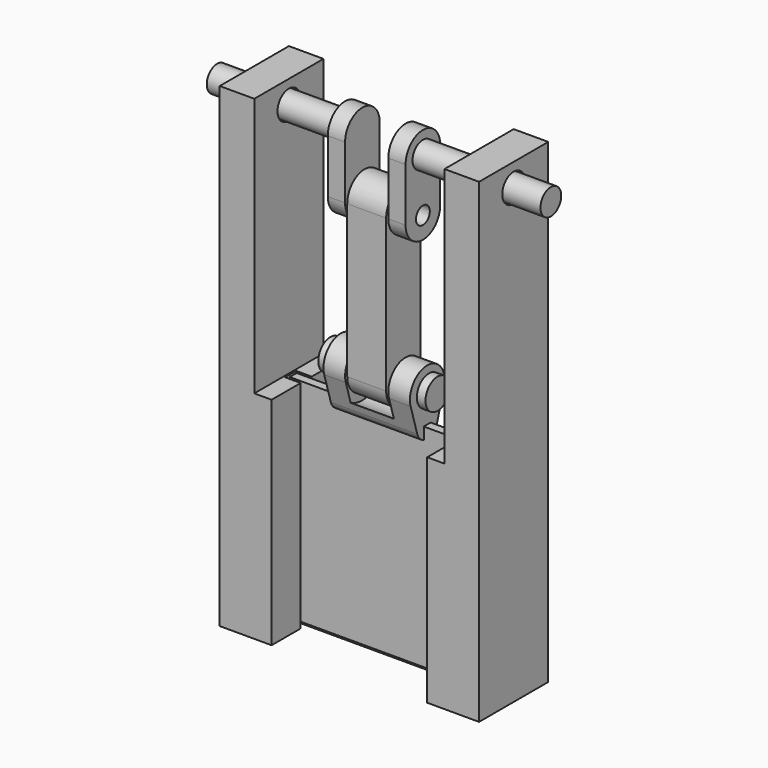
from build123d import *

# Parameters (mm, degrees)
F1_DEPTH  = 25
F0_W      = 21
F0_H      = 1
F2_SIZE   = 0.49999
F3_R      = 1
F4_DEPTH  = 5
F5_R      = 3.5
F5_R_2    = 1
F6_DEPTH  = 2.5
F7_R      = 0.8500000113
F8_DEPTH  = 5.2
F9_R      = 1.7489925994
F10_DEPTH = 1
F12_R     = 1
F12_R_2   = 1.1
F13_DEPTH = 2.25
F14_R     = 1
F15_DEPTH = 2.5
F16_R     = 1
F17_DEPTH = 2
F18_R     = 1.5
F19_DEPTH = 14.8
F21_W     = 10
F21_H     = 30
F21_R     = 1.65
F22_DEPTH = 4


# Not quite as in the source:
# - a fillet or chamfer is up to 0.001 mm smaller than in the source, because OpenCascade refuses the exact size


with BuildPart() as f1:
    # F0 (on Top) → F1 (new body)
    with BuildSketch(Plane.XY):
        Polygon((-9, 5), (-15, 5), (-15, -5), (-9, -5), (-9, -0.8), (-10.8, -0.8), (-10.8, 0.8), (-9, 0.8), align=None)
    extrude(amount=F1_DEPTH)

    # F23: F1b across plane


with BuildPart() as f1b:
    # F0 (on Top) → F1, piece 2 (new body)
    with BuildSketch(Plane.XY):
        Polygon((15, -5), (15, 5), (9, 5), (9, 0.8), (10.8, 0.8), (10.8, -0.8), (9, -0.8), (9, -5), align=None)
    extrude(amount=F1_DEPTH)

    # F21 (on face) → F22 (join)
    with BuildSketch(Plane.YZ.offset(15)):
        with Locations((0, 40)):
            Rectangle(F21_W, F21_H)
        with Locations((0, 52.3577854037)):
            Circle(F21_R, mode=Mode.SUBTRACT)
    extrude(amount=-F22_DEPTH)


with BuildPart() as f1c:
    # F0 (on Top) → F1, piece 3 (new body)
    with BuildSketch(Plane.XY):
        Rectangle(F0_W, F0_H)
    extrude(amount=F1_DEPTH)

    # F2 (size 0.5 in the source; OpenCascade refuses exactly that, so slightly less here)
    f2_edges = [f1c.edges().sort_by_distance(p)[0] for p in [
        (0, -0.5, 0),
        (0, 0.5, 0),
    ]]
    chamfer(f2_edges, length=F2_SIZE)

    # F3 (on Right) → F4 (join, symmetric)
    with BuildSketch(Plane.YZ):
        with BuildLine():
            Line((-2.3955912057, 27.8127531877), (-1.4373557878, 24.6019490366))
            ThreePointArc((-1.4373557878, 24.6019490366), (0, 23.5309109688), (1.4373557878, 24.6019490366))
            Line((1.4373557878, 24.6019490366), (2.3955912057, 27.8127531877))
            ThreePointArc((2.3955912057, 27.8127531877), (0, 31.0276956856), (-2.3955912057, 27.8127531877))
        make_face()
        with Locations((0, 28.5276956856)):
            Circle(F3_R, mode=Mode.SUBTRACT)
    extrude(amount=F4_DEPTH, both=True)

    # F5 (on Right) → F6 (cut, symmetric)
    with BuildSketch(Plane.YZ):
        with Locations((0, 28.5276956856)):
            Circle(F5_R)
        with Locations((0, 28.5276956856)):
            Circle(F5_R_2, mode=Mode.SUBTRACT)
    extrude(amount=F6_DEPTH, both=True, mode=Mode.SUBTRACT)


with BuildPart() as f8:
    # F7 (on Right) → F8 (new body)
    with BuildSketch(Plane.YZ):
        with Locations((0, 28.5276956856)):
            Circle(F7_R)
    extrude(amount=F8_DEPTH)

    # F9 (on face) → F10 (join)
    with BuildSketch(Plane.YZ.offset(5.2)):
        with Locations((0, 28.5276956856)):
            Circle(F9_R)
    extrude(amount=F10_DEPTH)

    # F11: F8 across plane


with BuildPart() as f8_1:
    add(f8.part)
    add(f8.part.mirror(Plane.YZ))


with BuildPart() as f13:
    # F12 (on Right) → F13 (new body, symmetric)
    with BuildSketch(Plane.YZ):
        with BuildLine():
            Line((-2.5, 46.1446046829), (-2.5, 28.5276956856))
            ThreePointArc((-2.5, 28.5276956856), (0, 26.0276956856), (2.5, 28.5276956856))
            Line((2.5, 28.5276956856), (2.5, 46.1446046829))
            ThreePointArc((2.5, 46.1446046829), (0, 48.6446046829), (-2.5, 46.1446046829))
        make_face()
        with Locations((0, 28.5276956856)):
            Circle(F12_R, mode=Mode.SUBTRACT)
        with Locations((0, 46.1446046829)):
            Circle(F12_R_2, mode=Mode.SUBTRACT)
    extrude(amount=F13_DEPTH, both=True)


with BuildPart() as f15:
    # F14 (on Right) → F15 (new body)
    with BuildSketch(Plane.YZ):
        with Locations((0, 46.1446046829)):
            Circle(F14_R)
    extrude(amount=F15_DEPTH)


with BuildPart() as f17:
    # F16 (on face) → F17 (new body)
    with BuildSketch(Plane.YZ.offset(2.5)):
        with BuildLine():
            Line((-2.5, 52.335832268), (-2.5, 46.1446046829))
            ThreePointArc((-2.5, 46.1446046829), (0, 43.6446046829), (2.5, 46.1446046829))
            Line((2.5, 46.1446046829), (2.5, 52.335832268))
            ThreePointArc((2.5, 52.335832268), (0, 54.835832268), (-2.5, 52.335832268))
        make_face()
        with Locations((0, 46.1446046829)):
            Circle(F16_R, mode=Mode.SUBTRACT)
    extrude(amount=F17_DEPTH)

    # F18 (on face) → F19 (join)
    with BuildSketch(Plane.YZ.offset(4.5)):
        with Locations((0, 52.335832268)):
            Circle(F18_R)
    extrude(amount=F19_DEPTH)


with BuildPart() as f20_1:
    # F20: instance of F17
    add(f17.part.mirror(Plane.YZ))


with BuildPart() as f1_1:
    add(f1.part)
    add(f1b.part.mirror(Plane.YZ))


solid = Compound([f1b.part, f1c.part, f8_1.part, f13.part, f15.part, f17.part, f20_1.part, f1_1.part])
